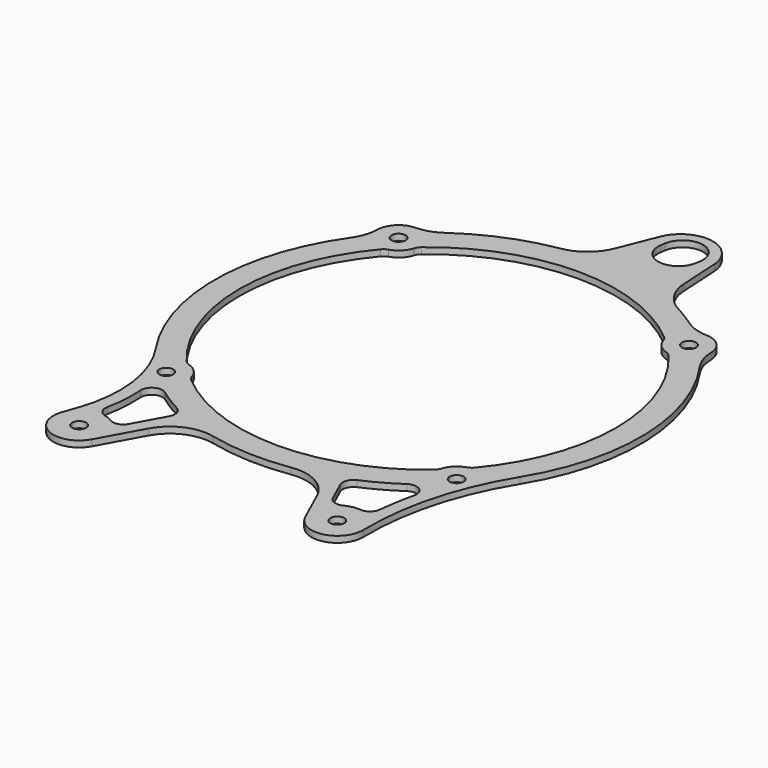
from build123d import *

# Parameters (mm, degrees)
F0_R     = 3.25
F1_DEPTH = 2.9


# Not quite as in the source:
# - ends of sketch curves that miss each other by under 0.0002 mm in the source are joined


with BuildPart() as f1:
    # F0 (on Top) → F1 (new body)
    with BuildSketch(Plane.XY):
        with BuildLine():
            ThreePointArc((-44.7213694768, -87.2696897378), (-35.3282259069, -78.6355727138), (-22.6261189451, -77.437406766))
            ThreePointArc((-22.6261189451, -77.437406766), (-3.9584138319, -79.9784717794), (14.8526419701, -78.9371528028))
            ThreePointArc((14.8526419701, -78.9371528028), (27.4184013914, -81.1464387638), (36.0916099164, -90.5034990376))
            Line((36.0916099164, -90.5034990376), (43.056946, -105.982018))
            ThreePointArc((43.056946, -105.982018), (56.6433108611, -112.762891287), (65.9972675289, -100.8015700101))
            ThreePointArc((65.9972675289, -100.8015700101), (70.3098677706, -65.4781038722), (84.4013998186, -32.8012868888))
            ThreePointArc((84.4013998186, -32.8012868888), (98.9543772418, 21.9475596078), (81.1058809507, 75.7123879655))
            ThreePointArc((81.1058809507, 75.7123879655), (78.4915241697, 80.9342205742), (77.4969704068, 86.68861601))
            ThreePointArc((77.4969704068, 86.68861601), (74.5710678119, 93.5134278119), (67.7462419947, 96.4393277843))
            ThreePointArc((67.7462419947, 96.4393277843), (61.9918305742, 97.4338841697), (56.7700159448, 100.0482399211))
            ThreePointArc((56.7700159448, 100.0482399211), (51.7741884012, 103.3250206324), (46.589782882, 106.2944757787))
            ThreePointArc((46.589782882, 106.2944757787), (39.1449717302, 113.1782098516), (36.0328533434, 122.8283870191))
            Line((36.0328533434, 122.8283870191), (34.976746, 141.777077))
            ThreePointArc((34.976746, 141.777077), (22.4266252093, 155.7447750088), (6.0736789634, 146.5152930146))
            Line((6.0736789634, 146.5152930146), (-0.977233, 128.895637))
            ThreePointArc((-0.977233, 128.895637), (-7.0076373704, 120.7442287718), (-16.2606700755, 116.5978324535))
            ThreePointArc((-16.2606700755, 116.5978324535), (-37.4411993299, 110.5892726198), (-56.7700327307, 100.0482376153))
            ThreePointArc((-56.7700327307, 100.0482376153), (-61.9918290994, 97.4338843258), (-67.7462240106, 96.4393304314))
            ThreePointArc((-67.7462240106, 96.4393304314), (-74.5710678119, 93.5134278119), (-77.4969677843, 86.6886019947))
            ThreePointArc((-77.4969677843, 86.6886019947), (-78.4915233258, 80.9342200994), (-81.1058789211, 75.7124059448))
            ThreePointArc((-81.1058789211, 75.7124059448), (-98.9973221942, 19.6705072268), (-81.9321709394, -36.6284899589))
            ThreePointArc((-81.9321709394, -36.6284899589), (-72.1246020826, -62.3015797591), (-74.7927308672, -89.6544180452))
            Line((-74.7927308672, -89.6544180452), (-77.359069, -97.188309))
            ThreePointArc((-77.359069, -97.188309), (-70.8446126339, -112.0362432093), (-55.4854090748, -106.8406649589))
            Line((-55.4854090748, -106.8406649589), (-44.7213694768, -87.2696897378))
        make_face()
        with Locations((-66, -101.05764)):
            Circle(F0_R, mode=Mode.SUBTRACT)
        with BuildLine():
            ThreePointArc((-52.5642634566, -89.0792787489), (-55.6931843813, -91.5103563164), (-59.6084751577, -90.9014372506))
            ThreePointArc((-59.6084751577, -90.9014372506), (-61.3402321592, -89.9993144635), (-63.1953610952, -89.3899923959))
            ThreePointArc((-63.1953610952, -89.3899923959), (-66.2453647932, -87.2123878479), (-66.9254446607, -83.5270150694))
            ThreePointArc((-66.9254446607, -83.5270150694), (-65.7348712362, -74.7077507104), (-65.7415821416, -65.8084890097))
            ThreePointArc((-65.7415821416, -65.8084890097), (-63.1835418456, -61.0980378443), (-57.8323762514, -61.4094713493))
            ThreePointArc((-57.8323762514, -61.4094713493), (-52.4648777131, -65.01260773), (-46.8736571173, -68.2577562181))
            ThreePointArc((-46.8736571173, -68.2577562181), (-44.4460535436, -71.2446768384), (-44.8599474566, -75.0713907489))
            Line((-44.8599474566, -75.0713907489), (-52.5642634566, -89.0792787489))
        make_face(mode=Mode.SUBTRACT)
        with Locations((-67.5, -48.55764)):
            Circle(F0_R, mode=Mode.SUBTRACT)
        with Locations((54, -101.05764)):
            Circle(F0_R, mode=Mode.SUBTRACT)
        with BuildLine():
            ThreePointArc((55.7668649484, -62.8565289244), (61.4137793469, -62.8660371217), (63.450485388, -68.1328730913))
            ThreePointArc((63.450485388, -68.1328730913), (61.7927741104, -76.349981087), (60.66398801, -84.656313001))
            ThreePointArc((60.66398801, -84.656313001), (58.8502515766, -88.0169614514), (55.1933120197, -89.1171158029))
            ThreePointArc((55.1933120197, -89.1171158029), (51.7212938161, -89.2759806038), (48.4404431818, -90.4231993478))
            ThreePointArc((48.4404431818, -90.4231993478), (44.4890186454, -90.7173209458), (41.5643552496, -88.0440028877))
            Line((41.5643552496, -88.0440028877), (37.204438, -78.355278))
            ThreePointArc((37.204438, -78.355278), (37.0976309763, -74.5077318057), (39.7561530447, -71.7243331019))
            ThreePointArc((39.7561530447, -71.7243331019), (47.9668749837, -67.6612132767), (55.7668649484, -62.8565289244))
        make_face(mode=Mode.SUBTRACT)
        with Locations((67.5, -48.55764)):
            Circle(F0_R, mode=Mode.SUBTRACT)
        with BuildLine():
            ThreePointArc((-57.9428097278, 83.4995499162), (-57.3338219129, 84.7875612773), (-56.3862887981, 85.8515257605))
            ThreePointArc((-56.3862887981, 85.8515257605), (-1.4091e-06, 106.44236), (56.3862897755, 85.8515247336))
            ThreePointArc((56.3862897755, 85.8515247336), (57.3338226492, 84.7875616758), (57.9428104466, 83.4995508296))
            ThreePointArc((57.9428104466, 83.4995508296), (60.4289318502, 79.371292526), (64.557188973, 76.8851709122))
            ThreePointArc((64.557188973, 76.8851709122), (65.8452017985, 76.276181568), (66.9091657605, 75.3286487981))
            ThreePointArc((66.9091657605, 75.3286487981), (87.5, 18.94236), (66.9091656417, -37.443928698))
            ThreePointArc((66.9091656417, -37.443928698), (65.8452017985, -38.391461568), (64.5571911108, -39.00044936))
            ThreePointArc((64.5571911108, -39.00044936), (60.4289318502, -41.486572526), (57.942810631, -45.6148298864))
            ThreePointArc((57.942810631, -45.6148298864), (57.3338226492, -46.9028416758), (56.3862897981, -47.9668057605))
            ThreePointArc((56.3862897981, -47.9668057605), (-1.4091e-06, -68.55764), (-56.3862919305, -47.9668029175))
            ThreePointArc((-56.3862919305, -47.9668029175), (-57.3338219129, -46.9028412773), (-57.9428097278, -45.6148299162))
            ThreePointArc((-57.9428097278, -45.6148299162), (-60.4289318502, -41.486572526), (-64.5571880596, -39.0004511935))
            ThreePointArc((-64.5571880596, -39.0004511935), (-65.8452006758, -38.3914616492), (-66.9091647605, -37.4439287981))
            ThreePointArc((-66.9091647605, -37.4439287981), (-87.5, 18.94236), (-66.9091638256, 75.328650853))
            ThreePointArc((-66.9091638256, 75.328650853), (-65.8452006758, 76.2761816492), (-64.5571898296, 76.8851694466))
            ThreePointArc((-64.5571898296, 76.8851694466), (-60.4289318502, 79.371292526), (-57.9428097278, 83.4995499162))
        make_face(mode=Mode.SUBTRACT)
        with Locations((-67.5, 86.44236)):
            Circle(F0_R, mode=Mode.SUBTRACT)
        with BuildLine():
            ThreePointArc((10.7869112155, 143.4660389647), (21.6986369647, 151.3040387845), (29.5366367845, 140.3923130353))
            Line((29.5366367845, 140.3923130353), (29.213074, 138.418678))
            ThreePointArc((29.213074, 138.418678), (18.3013640353, 130.5806802155), (10.4633642155, 141.4924059647))
            Line((10.4633642155, 141.4924059647), (10.7869112155, 143.4660389647))
        make_face(mode=Mode.SUBTRACT)
        with Locations((67.5, 86.44236)):
            Circle(F0_R, mode=Mode.SUBTRACT)
    extrude(amount=F1_DEPTH)


solid = f1.part
